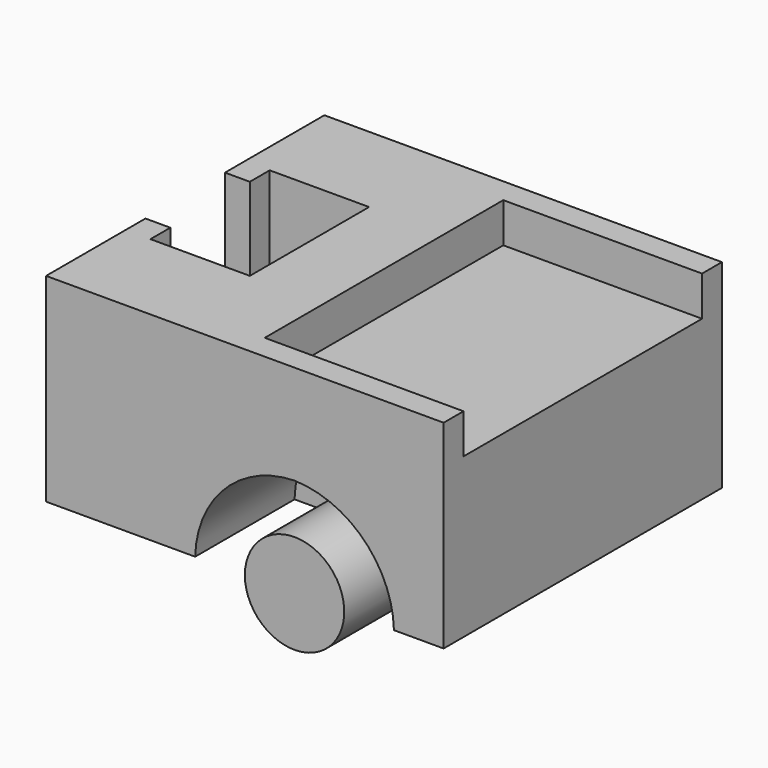
from build123d import *

# Parameters (mm, degrees)
F0_W          = 70
F0_H          = 40
F1_DEPTH      = 40
F1_DEPTH_BACK = 40
F2_W          = 40
F2_H          = 30
F3_DEPTH      = 8
F5_DEPTH      = 40
F6_W          = 40
F6_H          = 20
F7_DEPTH      = 25
F9_DEPTH      = 25
F10_W         = 80
F10_H         = 40
F11_DEPTH     = 35
F13_DEPTH     = 25
F14_T4_DEPTH  = 76.2347538298
F14_T9_DEPTH  = 76.2347538298
F14_T14_DEPTH = 76.2347538298
F14_T19_DEPTH = 76.2347538298
F15_W         = 5
F15_H         = 30
F16_DEPTH     = 10


# Not quite as in the source:
# - a fillet or chamfer that OpenCascade refuses, or shapes differently, is made with other operations: its cross-section is extruded or revolved along the edge and cut away or added


with BuildPart() as f1:
    # F0 (on Right) → F1 (new body, two sides)
    with BuildSketch(Plane.YZ) as f1_sk:
        Rectangle(F0_W, F0_H)
    extrude(amount=F1_DEPTH)
    extrude(f1_sk.sketch, amount=-F1_DEPTH_BACK)

    # F2 (on face) → F3 (cut)
    with BuildSketch(Plane.XY.offset(20)):
        with Locations((20, -15)):
            Rectangle(F2_W, F2_H)
        with Locations((20, 15)):
            Rectangle(F2_W, F2_H)
    extrude(amount=-F3_DEPTH, mode=Mode.SUBTRACT)

    # F4 (on face) → F5 (cut)
    with BuildSketch(Plane.XY.offset(20)):
        Polygon((-40, 10), (-40, 0), (-20, 0), (-20, 15), (-35, 15), (-35, 10), align=None)
        Polygon((-20, 0), (-40, 0), (-40, -10), (-35, -10), (-35, -15), (-20, -15), align=None)
    extrude(amount=-F5_DEPTH, mode=Mode.SUBTRACT)

    # F6 (on face) → F7 (cut)
    with BuildSketch(Plane.XZ.offset(35)):
        with Locations((10, -10)):
            Rectangle(F6_W, F6_H)
    extrude(amount=-F7_DEPTH, mode=Mode.SUBTRACT)

    # F8 (on face) → F9 (join)
    with BuildSketch(Plane.XZ.offset(10)):
        with BuildLine():
            Line((0, -20), (20, -20))
            ThreePointArc((20, -20), (10, -10), (0, -20))
        make_face()
        with BuildLine():
            ThreePointArc((0, -20), (10, -30), (20, -20))
            Line((20, -20), (0, -20))
        make_face()
    extrude(amount=F9_DEPTH)

    # F10 (on face) → F11 (cut)
    with BuildSketch(Plane(origin=(0, 35, 0), x_dir=(-1, 0, 0), z_dir=(0, 1, 0))):
        Rectangle(F10_W, F10_H)
    extrude(amount=-F11_DEPTH, mode=Mode.SUBTRACT)

    # F12: F1 across plane


with BuildPart() as f1_1:
    add(f1.part)
    add(f1.part.mirror(Plane.XZ))

    # F13 (add): a face of the model
    f13_faces = [f1_1.faces().sort_by_distance(p)[0] for p in [
        (10, -10, -24.2441318158),
    ]]
    extrude(f13_faces, amount=F13_DEPTH)

    # F14: fillet of radius 20.5 on 4 edges, made by hand


with BuildPart() as f14_tool2:
    # F14_s3 → F14_t4 (new body)
    with BuildSketch(Plane.XZ.offset(-35)):
        with BuildLine():
            ThreePointArc((30, -20), (23.8239195314, -5.8285992489), (9.5060984681, 0))
            Line((9.5060984681, 0), (30, 0))
            Line((30, 0), (30, -20))
        make_face()
    extrude(amount=F14_T4_DEPTH)

    split(bisect_by=Plane.XZ.offset(35), keep=Keep.BOTTOM)


with BuildPart() as f1_2:
    add(f1_1.part)

    # F14_t1: union F14_tool2
    add(f14_tool2.part)


with BuildPart() as f14_tool7:
    # F14_s8 → F14_t9 (new body)
    with BuildSketch(Plane.XZ.offset(-35)):
        with BuildLine():
            ThreePointArc((10.4939015319, 0), (-3.8239195314, -5.8285992489), (-10, -20))
            Line((-10, -20), (-10, 0))
            Line((-10, 0), (10.4939015319, 0))
        make_face()
    extrude(amount=F14_T9_DEPTH)

    split(bisect_by=Plane.XZ.offset(35), keep=Keep.BOTTOM)


with BuildPart() as f1_3:
    add(f1_2.part)

    # F14_t6: union F14_tool7
    add(f14_tool7.part)


with BuildPart() as f14_tool12:
    # F14_s13 → F14_t14 (new body)
    with BuildSketch(Plane.XZ.offset(35)):
        with BuildLine():
            ThreePointArc((30, -20), (23.8239195314, -5.8285992489), (9.5060984681, 0))
            Line((9.5060984681, 0), (30, 0))
            Line((30, 0), (30, -20))
        make_face()
    extrude(amount=-F14_T14_DEPTH)

    split(bisect_by=Plane.XZ.offset(-35), keep=Keep.TOP)


with BuildPart() as f1_4:
    add(f1_3.part)

    # F14_t11: union F14_tool12
    add(f14_tool12.part)


with BuildPart() as f14_tool17:
    # F14_s18 → F14_t19 (new body)
    with BuildSketch(Plane.XZ.offset(35)):
        with BuildLine():
            ThreePointArc((-10, -20), (-3.8239195314, -5.8285992489), (10.4939015319, 0))
            Line((10.4939015319, 0), (-10, 0))
            Line((-10, 0), (-10, -20))
        make_face()
    extrude(amount=-F14_T19_DEPTH)

    split(bisect_by=Plane.XZ.offset(-35), keep=Keep.TOP)


with BuildPart() as f1_5:
    add(f1_4.part)

    # F14_t16: union F14_tool17
    add(f14_tool17.part)

    # F15 (on face) → F16 (cut)
    with BuildSketch(Plane.XY.offset(20)):
        with Locations((-17.5, 0)):
            Rectangle(F15_W, F15_H)
    extrude(amount=-F16_DEPTH, mode=Mode.SUBTRACT)


solid = f1_5.part
